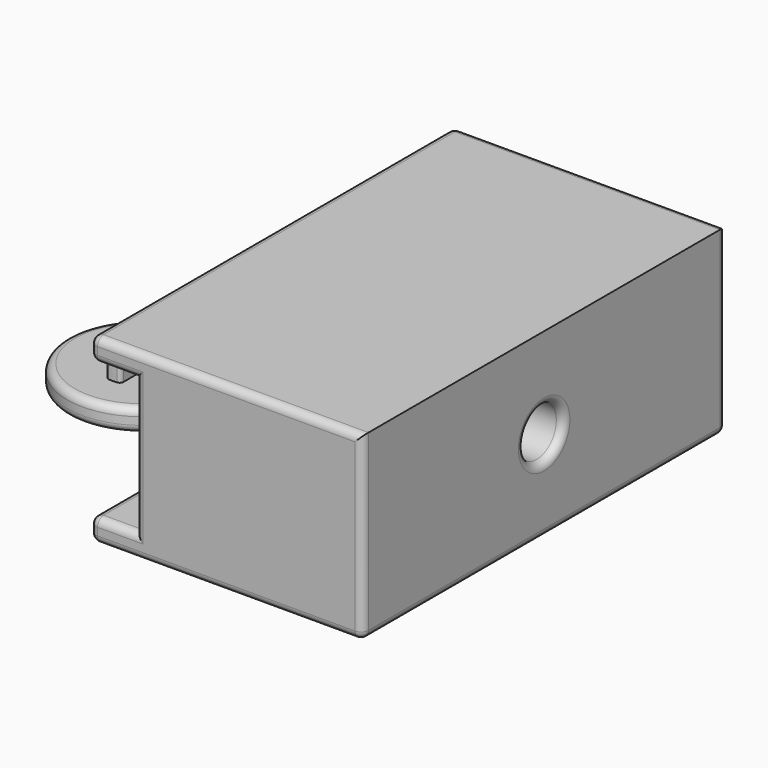
from build123d import *

# Parameters (mm, degrees)
F0_R     = 5
F1_DEPTH = 3
F3_DEPTH = 3
F4_W     = 30
F4_H     = 60
F5_DEPTH = 21
F6_W     = 60
F6_H     = 3
F7_DEPTH = 6
F8_R     = 3.25
F9_DEPTH = 30
F10_R    = 1
F11_R    = 0.5


# Not quite as in the source:
# - a feature names something its author has since deleted; it is built from what else it names


with BuildPart() as f1:
    # F0 (on Top) → F1 (new body)
    with BuildSketch(Plane.XY):
        with BuildLine():
            Line((17, 5), (8.6602540378, 5))
            ThreePointArc((8.6602540378, 5), (-10, 0), (8.6602540378, -5))
            Line((8.6602540378, -5), (17, -5))
            Line((17, -5), (17, -30))
            Line((17, -30), (53, -30))
            Line((53, -30), (53, 30))
            Line((53, 30), (17, 30))
            Line((17, 30), (17, 5))
        make_face()
        Circle(F0_R, mode=Mode.SUBTRACT)
        Circle(F0_R)
    extrude(amount=F1_DEPTH)

    # F2 (on face) → F3 (join)
    with BuildSketch(Plane.XY.offset(3)):
        with BuildLine():
            Line((1, -4.8989794856), (1, 4.8989794856))
            ThreePointArc((1, 4.8989794856), (0, 5), (-1, 4.8989794856))
            Line((-1, 4.8989794856), (-1, -4.8989794856))
            ThreePointArc((-1, -4.8989794856), (0, -5), (1, -4.8989794856))
        make_face()
    extrude(amount=F3_DEPTH)

    # F4 (on face) → F5 (join)
    with BuildSketch(Plane.XY.offset(3)):
        with Locations((38, 0)):
            Rectangle(F4_W, F4_H)
    extrude(amount=F5_DEPTH)

    # F6 (on face) → F7 (join)
    with BuildSketch(Plane(origin=(23, 0, 0), x_dir=(0, -1, 0), z_dir=(-1, 0, 0))):
        with Locations((0, 22.5)):
            Rectangle(F6_W, F6_H)
    extrude(amount=F7_DEPTH)

    # F8 (on face) → F9 (cut)
    with BuildSketch(Plane(origin=(23, 0, 0), x_dir=(0, -1, 0), z_dir=(-1, 0, 0))):
        with Locations((0, 12)):
            Circle(F8_R)
    extrude(amount=-F9_DEPTH, mode=Mode.SUBTRACT)

    # F10
    f10_edges = [f1.edges().sort_by_distance(p)[0] for p in [
        (17, -30, 1.5),
        (17, 30, 1.5),
        (23, 3.25, 12),
        (12.830127, -5, 3),
        (-10, 0, 3),
        (12.830127, 5, 3),
        (35, 30, 0),
        (53, 30, 12),
        (17, 17.5, 0),
        (12.830127, 5, 0),
        (-10, 0, 0),
        (12.830127, -5, 0),
        (17, -17.5, 0),
        (53, 0, 0),
        (35, -30, 0),
        (53, -30, 12),
        (53, 3.25, 12),
        (23, -30, 12),
        (23, 30, 12),
        (20, 30, 21),
        (17, 0, 21),
        (17, 30, 22.5),
        (17, 0, 24),
        (35, 30, 24),
        (35, -30, 24),
        (17, -30, 22.5),
        (20, -30, 21),
        (20, -30, 3),
        (17, -17.5, 3),
        (17, 17.5, 3),
    ]]
    fillet(f10_edges, radius=F10_R)

    # F11
    f11_edges = [f1.edges().sort_by_distance(p)[0] for p in [
        (0, -5, 6),
        (0, 5, 6),
        (-1, -4.898979, 4.5),
        (1, -4.898979, 4.5),
        (1, 4.898979, 4.5),
        (-1, 4.898979, 4.5),
        (-1, 0, 6),
        (1, 0, 6),
    ]]
    fillet(f11_edges, radius=F11_R)


solid = f1.part
